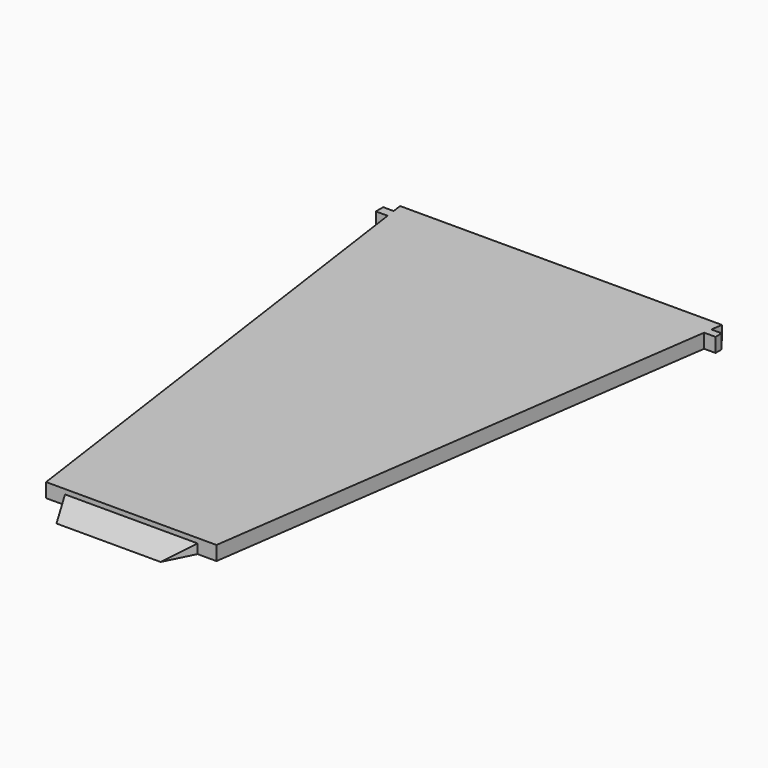
from build123d import *

# Parameters (mm, degrees)
F1_DEPTH = 1.5
F3_DEPTH = 1
F4_SIZE2 = 2.99999
F4_SIZE  = 0.99999
F5_W     = 2.5577563792
F5_H     = 0.9680986404
F5_W_2   = 3.2131588086
F5_H_2   = 0.8198879659
F6_DEPTH = 1.5
F7_DEPTH = 1.5


# Not quite as in the source:
# - a fillet or chamfer is up to 0.001 mm smaller than in the source, because OpenCascade refuses the exact size


with BuildPart() as f1:
    # F0 (on Top) → F1 (new body)
    with BuildSketch(Plane.XY):
        Polygon((17, 27.609485096), (0, 27.609485096), (0, -29.140514904), (7, -29.140514904), (9, -29.140514904), align=None)
        Polygon((0, -29.140514904), (0, 27.609485096), (-17, 27.609485096), (-9, -29.140514904), (-7, -29.140514904), align=None)
    extrude(amount=F1_DEPTH)

    # F5 (on face) → F6 (join)
    with BuildSketch(Plane(origin=(0, 0, 0), x_dir=(1, 0, 0), z_dir=(0, 0, -1))):
        with Locations((-16.6856339201, -26.0949004441)):
            Rectangle(F5_W, F5_H)
        with Locations((16.3177815266, -26.0207951069)):
            Rectangle(F5_W_2, F5_H_2)
    extrude(amount=-F6_DEPTH)

    # F5 (on face) → F7 (join)
    with BuildSketch(Plane(origin=(0, 0, 0), x_dir=(1, 0, 0), z_dir=(0, 0, -1))):
        with Locations((-16.6856339201, -26.0949004441)):
            Rectangle(F5_W, F5_H)
        with Locations((16.3177815266, -26.0207951069)):
            Rectangle(F5_W_2, F5_H_2)
    extrude(amount=-F7_DEPTH)


with BuildPart() as f3:
    # F2 (on face) → F3 (new body)
    with BuildSketch(Plane(origin=(0, 0, 0), x_dir=(1, 0, 0), z_dir=(0, 0, -1))):
        Polygon((-5.5, 29.140514904), (0, 29.140514904), (5.5, 29.140514904), (7, 29.140514904), (5.5, 32.140514904), (0, 32.140514904), (-5.5, 32.140514904), align=None)
        Polygon((-7, 29.140514904), (-5.5, 29.140514904), (-5.5, 32.140514904), align=None)
    extrude(amount=-F3_DEPTH)

    # F4 (size 1 and 3 in the source; OpenCascade refuses exactly that, so slightly less here)
    f4_edges = [f3.edges().sort_by_distance(p)[0] for p in [
        (0, -32.140515, 1),
    ]]
    chamfer(f4_edges, length=F4_SIZE, length2=F4_SIZE2)


solid = Compound([f1.part, f3.part])
